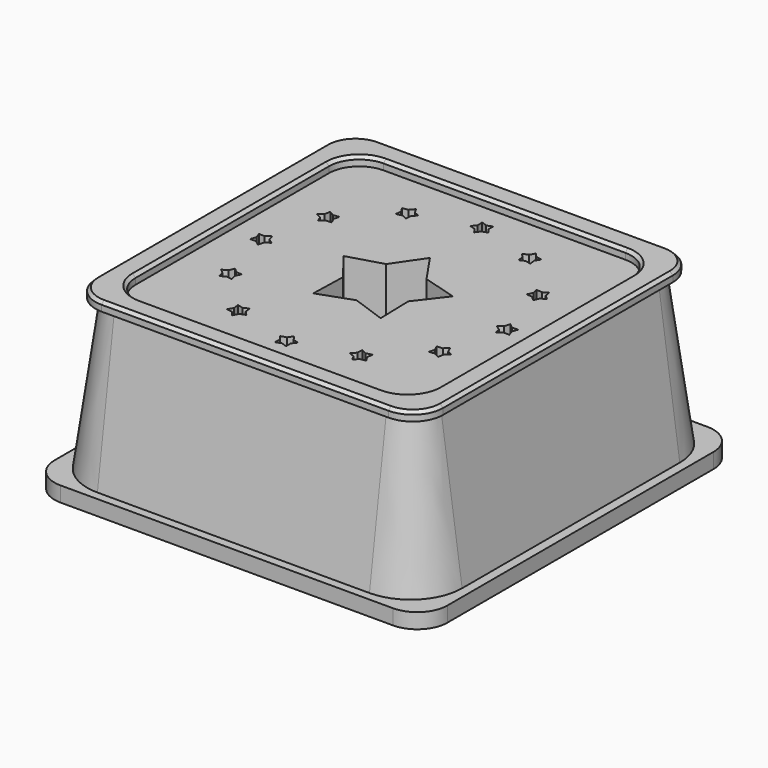
from build123d import *

# Parameters (mm, degrees)
F1_DEPTH = 50
F2_DEPTH = 3
F3_SIZE2 = 1
F3_SIZE  = 1
F4_START = -50
F4_DEPTH = 5
F5_DEPTH = 50
F5_TAPER = -8
F6_START = -25
F6_DEPTH = 25
F7_START = -10
F7_DEPTH = 40


with BuildPart() as f1:
    # F0 (on Top) → F1 (new body)
    with BuildSketch(Plane.XY):
        with BuildLine():
            Line((-39.9938075139, -50.2834277693), (40.0061924861, -50.2834277693))
            ThreePointArc((40.0061924861, -50.2834277693), (47.077260298, -47.3544955812), (50.0061924861, -40.2834277693))
            Line((50.0061924861, -40.2834277693), (50.0061924861, 39.7165722307))
            ThreePointArc((50.0061924861, 39.7165722307), (47.077260298, 46.7876400425), (40.0061924861, 49.7165722307))
            Line((40.0061924861, 49.7165722307), (-39.9938075139, 49.7165722307))
            ThreePointArc((-39.9938075139, 49.7165722307), (-47.0648753257, 46.7876400425), (-49.9938075139, 39.7165722307))
            Line((-49.9938075139, 39.7165722307), (-49.9938075139, -40.2834277693))
            ThreePointArc((-49.9938075139, -40.2834277693), (-47.0648753257, -47.3544955812), (-39.9938075139, -50.2834277693))
        make_face()
        Polygon((-23.019393146, -36.2108037162), (-21.9985903732, -34.5499172895), (-22.2534069929, -32.6163814143), (-20.3583647293, -33.0739804117), (-18.5998738672, -32.2323796091), (-18.449476111, -34.1760777694), (-17.1056626227, -35.5884330122), (-18.9077539612, -36.3321055417), (-19.835722413, -38.0465898886), (-21.0998738672, -36.562506628), align=None, mode=Mode.SUBTRACT)
        Polygon((-38.0407811023, -19.8497793366), (-36.3262967554, -18.9218108848), (-35.5802064838, -17.1199113878), (-34.167851241, -18.4637248762), (-32.2241530807, -18.6141226323), (-33.0657538833, -20.3726134945), (-32.6081548859, -22.2676557581), (-34.5406480297, -22.0106493915), (-36.2015344564, -23.0314521644), (-36.5542800996, -21.1141226323), align=None, mode=Mode.SUBTRACT)
        Polygon((1.8450554322, -42.8671745774), (0.0082265284, -42.2139964995), (-1.8299773861, -42.8691724827), (-1.7763794659, -40.920401258), (-2.9638250695, -39.3733183808), (-1.0938708292, -38.8220896055), (0.0082265284, -37.2139964995), (1.1103238861, -38.8220896055), (2.9802781263, -39.3733183808), (1.791457512, -40.9184033527), align=None, mode=Mode.SUBTRACT)
        Polygon((19.8497793366, -38.0407811023), (18.9218108848, -36.3262967554), (17.1199113878, -35.5802064838), (18.4637248762, -34.167851241), (18.6141226323, -32.2241530807), (20.3726134945, -33.0657538833), (22.2676557581, -32.6081548859), (22.0106493915, -34.5406480297), (23.0314521644, -36.2015344564), (21.1141226323, -36.5542800996), align=None, mode=Mode.SUBTRACT)
        Polygon((36.2108037162, -23.019393146), (34.5499172895, -21.9985903732), (32.6163814143, -22.2534069929), (33.0739804117, -20.3583647293), (32.2323796091, -18.5998738672), (34.1760777694, -18.449476111), (35.5884330122, -17.1056626227), (36.3321055417, -18.9077539612), (38.0465898886, -19.835722413), (36.562506628, -21.0998738672), align=None, mode=Mode.SUBTRACT)
        Polygon((-42.8691724827, 1.8299773861), (-40.920401258, 1.7763794659), (-39.3733183808, 2.9638250695), (-38.8220896055, 1.0938708292), (-37.2139964995, -0.0082265284), (-38.8220896055, -1.1103238861), (-39.3733183808, -2.9802781263), (-40.9184033527, -1.791457512), (-42.8671745774, -1.8450554322), (-42.2139964995, -0.0082265284), align=None, mode=Mode.SUBTRACT)
        Polygon((-36.2108037162, 23.019393146), (-34.5499172895, 21.9985903732), (-32.6163814143, 22.2534069929), (-33.0739804117, 20.3583647293), (-32.2323796091, 18.5998738672), (-34.1760777694, 18.449476111), (-35.5884330122, 17.1056626227), (-36.3321055417, 18.9077539612), (-38.0465898886, 19.835722413), (-36.562506628, 21.0998738672), align=None, mode=Mode.SUBTRACT)
        Polygon((-10.8260939496, -3.5273158742), (-18.037479796, 5.8451695652), (-6.6943373747, 9.1889233161), (-0.0090148032, 18.9436160971), (6.6763077683, 9.1889233161), (18.0194501896, 5.8451695652), (10.8080643433, -3.5273158742), (11.1331893274, -15.3485621233), (-0.0090148032, -11.3863839029), (-11.1512189337, -15.3485621233), align=None, mode=Mode.SUBTRACT)
        Polygon((-19.8497793366, 38.0407811023), (-18.9218108848, 36.3262967554), (-17.1199113878, 35.5802064838), (-18.4637248762, 34.167851241), (-18.6141226323, 32.2241530807), (-20.3726134945, 33.0657538833), (-22.2676557581, 32.6081548859), (-22.0106493915, 34.5406480297), (-23.0314521644, 36.2015344564), (-21.1141226323, 36.5542800996), align=None, mode=Mode.SUBTRACT)
        Polygon((1.8299773861, 42.8691724827), (1.7763794659, 40.920401258), (2.9638250695, 39.3733183808), (1.0938708292, 38.8220896055), (-0.0082265284, 37.2139964995), (-1.1103238861, 38.8220896055), (-2.9802781263, 39.3733183808), (-1.791457512, 40.9184033527), (-1.8450554322, 42.8671745774), (-0.0082265284, 42.2139964995), align=None, mode=Mode.SUBTRACT)
        Polygon((42.8691724827, -1.8299773861), (40.920401258, -1.7763794659), (39.3733183808, -2.9638250695), (38.8220896055, -1.0938708292), (37.2139964995, 0.0082265284), (38.8220896055, 1.1103238861), (39.3733183808, 2.9802781263), (40.9184033527, 1.791457512), (42.8671745774, 1.8450554322), (42.2139964995, 0.0082265284), align=None, mode=Mode.SUBTRACT)
        Polygon((38.0407811023, 19.8497793366), (36.3262967554, 18.9218108848), (35.5802064838, 17.1199113878), (34.167851241, 18.4637248762), (32.2241530807, 18.6141226323), (33.0657538833, 20.3726134945), (32.6081548859, 22.2676557581), (34.5406480297, 22.0106493915), (36.2015344564, 23.0314521644), (36.5542800996, 21.1141226323), align=None, mode=Mode.SUBTRACT)
        Polygon((23.019393146, 36.2108037162), (21.9985903732, 34.5499172895), (22.2534069929, 32.6163814143), (20.3583647293, 33.0739804117), (18.5998738672, 32.2323796091), (18.449476111, 34.1760777694), (17.1056626227, 35.5884330122), (18.9077539612, 36.3321055417), (19.835722413, 38.0465898886), (21.0998738672, 36.562506628), align=None, mode=Mode.SUBTRACT)
    extrude(amount=-F1_DEPTH)

    # F0 (on Top) → F5 (join)
    with BuildSketch(Plane.XY):
        with BuildLine():
            Line((-45.0879924628, -55.17156791), (44.9120075372, -55.17156791))
            ThreePointArc((44.9120075372, -55.17156791), (51.9830753491, -52.2426357219), (54.9120075372, -45.17156791))
            Line((54.9120075372, -45.17156791), (54.9120075372, 44.82843209))
            ThreePointArc((54.9120075372, 44.82843209), (51.9830753491, 51.8994999019), (44.9120075372, 54.82843209))
            Line((44.9120075372, 54.82843209), (-45.0879924628, 54.82843209))
            ThreePointArc((-45.0879924628, 54.82843209), (-52.1590602747, 51.8994999019), (-55.0879924628, 44.82843209))
            Line((-55.0879924628, 44.82843209), (-55.0879924628, -45.17156791))
            ThreePointArc((-55.0879924628, -45.17156791), (-52.1590602747, -52.2426357219), (-45.0879924628, -55.17156791))
        make_face()
        with BuildLine():
            ThreePointArc((50.0061924861, -40.2834277693), (47.077260298, -47.3544955812), (40.0061924861, -50.2834277693))
            Line((40.0061924861, -50.2834277693), (-39.9938075139, -50.2834277693))
            ThreePointArc((-39.9938075139, -50.2834277693), (-47.0648753257, -47.3544955812), (-49.9938075139, -40.2834277693))
            Line((-49.9938075139, -40.2834277693), (-49.9938075139, 39.7165722307))
            ThreePointArc((-49.9938075139, 39.7165722307), (-47.0648753257, 46.7876400425), (-39.9938075139, 49.7165722307))
            Line((-39.9938075139, 49.7165722307), (40.0061924861, 49.7165722307))
            ThreePointArc((40.0061924861, 49.7165722307), (47.077260298, 46.7876400425), (50.0061924861, 39.7165722307))
            Line((50.0061924861, 39.7165722307), (50.0061924861, -40.2834277693))
        make_face(mode=Mode.SUBTRACT)
    extrude(amount=-F5_DEPTH, taper=F5_TAPER)

    # F0 (on Top) → F6 (join)
    with BuildSketch(Plane.XY.offset(F6_START)):
        Polygon((-6.6943373747, 9.1889233161), (-18.037479796, 5.8451695652), (-10.8260939496, -3.5273158742), (-11.1512189337, -15.3485621233), (-0.0090148032, -11.3863839029), (11.1331893274, -15.3485621233), (10.8080643433, -3.5273158742), (18.0194501896, 5.8451695652), (6.6763077683, 9.1889233161), (-0.0090148032, 18.9436160971), align=None)
    extrude(amount=-F6_DEPTH)

    # F0 (on Top) → F7 (join)
    with BuildSketch(Plane.XY.offset(F7_START)):
        Polygon((32.6163814143, -22.2534069929), (34.5499172895, -21.9985903732), (36.2108037162, -23.019393146), (36.562506628, -21.0998738672), (38.0465898886, -19.835722413), (36.3321055417, -18.9077539612), (35.5884330122, -17.1056626227), (34.1760777694, -18.449476111), (32.2323796091, -18.5998738672), (33.0739804117, -20.3583647293), align=None)
        Polygon((39.3733183808, -2.9638250695), (40.920401258, -1.7763794659), (42.8691724827, -1.8299773861), (42.2139964995, 0.0082265284), (42.8671745774, 1.8450554322), (40.9184033527, 1.791457512), (39.3733183808, 2.9802781263), (38.8220896055, 1.1103238861), (37.2139964995, 0.0082265284), (38.8220896055, -1.0938708292), align=None)
        Polygon((17.1199113878, -35.5802064838), (18.9218108848, -36.3262967554), (19.8497793366, -38.0407811023), (21.1141226323, -36.5542800996), (23.0314521644, -36.2015344564), (22.0106493915, -34.5406480297), (22.2676557581, -32.6081548859), (20.3726134945, -33.0657538833), (18.6141226323, -32.2241530807), (18.4637248762, -34.167851241), align=None)
        Polygon((-1.8299773861, -42.8691724827), (0.0082265284, -42.2139964995), (1.8450554322, -42.8671745774), (1.791457512, -40.9184033527), (2.9802781263, -39.3733183808), (1.1103238861, -38.8220896055), (0.0082265284, -37.2139964995), (-1.0938708292, -38.8220896055), (-2.9638250695, -39.3733183808), (-1.7763794659, -40.920401258), align=None)
        Polygon((-22.2534069929, -32.6163814143), (-21.9985903732, -34.5499172895), (-23.019393146, -36.2108037162), (-21.0998738672, -36.562506628), (-19.835722413, -38.0465898886), (-18.9077539612, -36.3321055417), (-17.1056626227, -35.5884330122), (-18.449476111, -34.1760777694), (-18.5998738672, -32.2323796091), (-20.3583647293, -33.0739804117), align=None)
        Polygon((-35.5802064838, -17.1199113878), (-36.3262967554, -18.9218108848), (-38.0407811023, -19.8497793366), (-36.5542800996, -21.1141226323), (-36.2015344564, -23.0314521644), (-34.5406480297, -22.0106493915), (-32.6081548859, -22.2676557581), (-33.0657538833, -20.3726134945), (-32.2241530807, -18.6141226323), (-34.167851241, -18.4637248762), align=None)
        Polygon((-39.3733183808, 2.9638250695), (-40.920401258, 1.7763794659), (-42.8691724827, 1.8299773861), (-42.2139964995, -0.0082265284), (-42.8671745774, -1.8450554322), (-40.9184033527, -1.791457512), (-39.3733183808, -2.9802781263), (-38.8220896055, -1.1103238861), (-37.2139964995, -0.0082265284), (-38.8220896055, 1.0938708292), align=None)
        Polygon((-17.1199113878, 35.5802064838), (-18.9218108848, 36.3262967554), (-19.8497793366, 38.0407811023), (-21.1141226323, 36.5542800996), (-23.0314521644, 36.2015344564), (-22.0106493915, 34.5406480297), (-22.2676557581, 32.6081548859), (-20.3726134945, 33.0657538833), (-18.6141226323, 32.2241530807), (-18.4637248762, 34.167851241), align=None)
        Polygon((2.9638250695, 39.3733183808), (1.7763794659, 40.920401258), (1.8299773861, 42.8691724827), (-0.0082265284, 42.2139964995), (-1.8450554322, 42.8671745774), (-1.791457512, 40.9184033527), (-2.9802781263, 39.3733183808), (-1.1103238861, 38.8220896055), (-0.0082265284, 37.2139964995), (1.0938708292, 38.8220896055), align=None)
        Polygon((22.2534069929, 32.6163814143), (21.9985903732, 34.5499172895), (23.019393146, 36.2108037162), (21.0998738672, 36.562506628), (19.835722413, 38.0465898886), (18.9077539612, 36.3321055417), (17.1056626227, 35.5884330122), (18.449476111, 34.1760777694), (18.5998738672, 32.2323796091), (20.3583647293, 33.0739804117), align=None)
        Polygon((35.5802064838, 17.1199113878), (36.3262967554, 18.9218108848), (38.0407811023, 19.8497793366), (36.5542800996, 21.1141226323), (36.2015344564, 23.0314521644), (34.5406480297, 22.0106493915), (32.6081548859, 22.2676557581), (33.0657538833, 20.3726134945), (32.2241530807, 18.6141226323), (34.167851241, 18.4637248762), align=None)
        Polygon((-32.6163814143, 22.2534069929), (-34.5499172895, 21.9985903732), (-36.2108037162, 23.019393146), (-36.562506628, 21.0998738672), (-38.0465898886, 19.835722413), (-36.3321055417, 18.9077539612), (-35.5884330122, 17.1056626227), (-34.1760777694, 18.449476111), (-32.2323796091, 18.5998738672), (-33.0739804117, 20.3583647293), align=None)
    extrude(amount=-F7_DEPTH)


with BuildPart() as f2:
    # F0 (on Top) → F2 (new body)
    with BuildSketch(Plane.XY):
        with BuildLine():
            Line((-47.4867287506, -57.5086505979), (47.5132712494, -57.5086505979))
            ThreePointArc((47.5132712494, -57.5086505979), (54.5843390612, -54.5797184098), (57.5132712494, -47.5086505979))
            Line((57.5132712494, -47.5086505979), (57.5132712494, 47.4913494021))
            ThreePointArc((57.5132712494, 47.4913494021), (54.5843390612, 54.5624172139), (47.5132712494, 57.4913494021))
            Line((47.5132712494, 57.4913494021), (-47.4867287506, 57.4913494021))
            ThreePointArc((-47.4867287506, 57.4913494021), (-54.5577965625, 54.5624172139), (-57.4867287506, 47.4913494021))
            Line((-57.4867287506, 47.4913494021), (-57.4867287506, -47.5086505979))
            ThreePointArc((-57.4867287506, -47.5086505979), (-54.5577965625, -54.5797184098), (-47.4867287506, -57.5086505979))
        make_face()
        with BuildLine():
            ThreePointArc((54.9120075372, -45.17156791), (51.9830753491, -52.2426357219), (44.9120075372, -55.17156791))
            Line((44.9120075372, -55.17156791), (-45.0879924628, -55.17156791))
            ThreePointArc((-45.0879924628, -55.17156791), (-52.1590602747, -52.2426357219), (-55.0879924628, -45.17156791))
            Line((-55.0879924628, -45.17156791), (-55.0879924628, 44.82843209))
            ThreePointArc((-55.0879924628, 44.82843209), (-52.1590602747, 51.8994999019), (-45.0879924628, 54.82843209))
            Line((-45.0879924628, 54.82843209), (44.9120075372, 54.82843209))
            ThreePointArc((44.9120075372, 54.82843209), (51.9830753491, 51.8994999019), (54.9120075372, 44.82843209))
            Line((54.9120075372, 44.82843209), (54.9120075372, -45.17156791))
        make_face(mode=Mode.SUBTRACT)
        with BuildLine():
            Line((-45.0879924628, -55.17156791), (44.9120075372, -55.17156791))
            ThreePointArc((44.9120075372, -55.17156791), (51.9830753491, -52.2426357219), (54.9120075372, -45.17156791))
            Line((54.9120075372, -45.17156791), (54.9120075372, 44.82843209))
            ThreePointArc((54.9120075372, 44.82843209), (51.9830753491, 51.8994999019), (44.9120075372, 54.82843209))
            Line((44.9120075372, 54.82843209), (-45.0879924628, 54.82843209))
            ThreePointArc((-45.0879924628, 54.82843209), (-52.1590602747, 51.8994999019), (-55.0879924628, 44.82843209))
            Line((-55.0879924628, 44.82843209), (-55.0879924628, -45.17156791))
            ThreePointArc((-55.0879924628, -45.17156791), (-52.1590602747, -52.2426357219), (-45.0879924628, -55.17156791))
        make_face()
        with BuildLine():
            ThreePointArc((50.0061924861, -40.2834277693), (47.077260298, -47.3544955812), (40.0061924861, -50.2834277693))
            Line((40.0061924861, -50.2834277693), (-39.9938075139, -50.2834277693))
            ThreePointArc((-39.9938075139, -50.2834277693), (-47.0648753257, -47.3544955812), (-49.9938075139, -40.2834277693))
            Line((-49.9938075139, -40.2834277693), (-49.9938075139, 39.7165722307))
            ThreePointArc((-49.9938075139, 39.7165722307), (-47.0648753257, 46.7876400425), (-39.9938075139, 49.7165722307))
            Line((-39.9938075139, 49.7165722307), (40.0061924861, 49.7165722307))
            ThreePointArc((40.0061924861, 49.7165722307), (47.077260298, 46.7876400425), (50.0061924861, 39.7165722307))
            Line((50.0061924861, 39.7165722307), (50.0061924861, -40.2834277693))
        make_face(mode=Mode.SUBTRACT)
    extrude(amount=F2_DEPTH)

    # F3
    f3_edges = [f2.edges().sort_by_distance(p)[0] for p in [
        (47.07726, -47.354496, 3),
        (0.006192, -50.283428, 3),
        (-47.064875, -47.354496, 3),
        (-49.993808, -0.283428, 3),
        (-47.064875, 46.78764, 3),
        (0.006192, 49.716572, 3),
        (47.07726, 46.78764, 3),
        (50.006192, -0.283428, 3),
        (0.013271, -57.508651, 3),
        (54.584339, -54.579718, 3),
        (57.513271, -0.008651, 3),
        (54.584339, 54.562417, 3),
        (0.013271, 57.491349, 3),
        (-54.557797, 54.562417, 3),
        (-57.486729, -0.008651, 3),
        (-54.557797, -54.579718, 3),
    ]]
    chamfer(f3_edges, length=F3_SIZE, length2=F3_SIZE2)


with BuildPart() as f4:
    # F0 (on Top) → F4 (new body)
    with BuildSketch(Plane.XY.offset(F4_START)):
        with BuildLine():
            Line((-54.9997077189, -65.0502125877), (55.0002922811, -65.0502125877))
            ThreePointArc((55.0002922811, -65.0502125877), (62.0713600929, -62.1212803995), (65.0002922811, -55.0502125877))
            Line((65.0002922811, -55.0502125877), (65.0002922811, 54.9497874123))
            ThreePointArc((65.0002922811, 54.9497874123), (62.0713600929, 62.0208552242), (55.0002922811, 64.9497874123))
            Line((55.0002922811, 64.9497874123), (-54.9997077189, 64.9497874123))
            ThreePointArc((-54.9997077189, 64.9497874123), (-62.0707755308, 62.0208552242), (-64.9997077189, 54.9497874123))
            Line((-64.9997077189, 54.9497874123), (-64.9997077189, -55.0502125877))
            ThreePointArc((-64.9997077189, -55.0502125877), (-62.0707755308, -62.1212803995), (-54.9997077189, -65.0502125877))
        make_face()
        with BuildLine():
            ThreePointArc((57.5132712494, -47.5086505979), (54.5843390612, -54.5797184098), (47.5132712494, -57.5086505979))
            Line((47.5132712494, -57.5086505979), (-47.4867287506, -57.5086505979))
            ThreePointArc((-47.4867287506, -57.5086505979), (-54.5577965625, -54.5797184098), (-57.4867287506, -47.5086505979))
            Line((-57.4867287506, -47.5086505979), (-57.4867287506, 47.4913494021))
            ThreePointArc((-57.4867287506, 47.4913494021), (-54.5577965625, 54.5624172139), (-47.4867287506, 57.4913494021))
            Line((-47.4867287506, 57.4913494021), (47.5132712494, 57.4913494021))
            ThreePointArc((47.5132712494, 57.4913494021), (54.5843390612, 54.5624172139), (57.5132712494, 47.4913494021))
            Line((57.5132712494, 47.4913494021), (57.5132712494, -47.5086505979))
        make_face(mode=Mode.SUBTRACT)
        with BuildLine():
            Line((-47.4867287506, -57.5086505979), (47.5132712494, -57.5086505979))
            ThreePointArc((47.5132712494, -57.5086505979), (54.5843390612, -54.5797184098), (57.5132712494, -47.5086505979))
            Line((57.5132712494, -47.5086505979), (57.5132712494, 47.4913494021))
            ThreePointArc((57.5132712494, 47.4913494021), (54.5843390612, 54.5624172139), (47.5132712494, 57.4913494021))
            Line((47.5132712494, 57.4913494021), (-47.4867287506, 57.4913494021))
            ThreePointArc((-47.4867287506, 57.4913494021), (-54.5577965625, 54.5624172139), (-57.4867287506, 47.4913494021))
            Line((-57.4867287506, 47.4913494021), (-57.4867287506, -47.5086505979))
            ThreePointArc((-57.4867287506, -47.5086505979), (-54.5577965625, -54.5797184098), (-47.4867287506, -57.5086505979))
        make_face()
        with BuildLine():
            ThreePointArc((54.9120075372, -45.17156791), (51.9830753491, -52.2426357219), (44.9120075372, -55.17156791))
            Line((44.9120075372, -55.17156791), (-45.0879924628, -55.17156791))
            ThreePointArc((-45.0879924628, -55.17156791), (-52.1590602747, -52.2426357219), (-55.0879924628, -45.17156791))
            Line((-55.0879924628, -45.17156791), (-55.0879924628, 44.82843209))
            ThreePointArc((-55.0879924628, 44.82843209), (-52.1590602747, 51.8994999019), (-45.0879924628, 54.82843209))
            Line((-45.0879924628, 54.82843209), (44.9120075372, 54.82843209))
            ThreePointArc((44.9120075372, 54.82843209), (51.9830753491, 51.8994999019), (54.9120075372, 44.82843209))
            Line((54.9120075372, 44.82843209), (54.9120075372, -45.17156791))
        make_face(mode=Mode.SUBTRACT)
    extrude(amount=-F4_DEPTH)


solid = Compound([f1.part, f2.part, f4.part])
